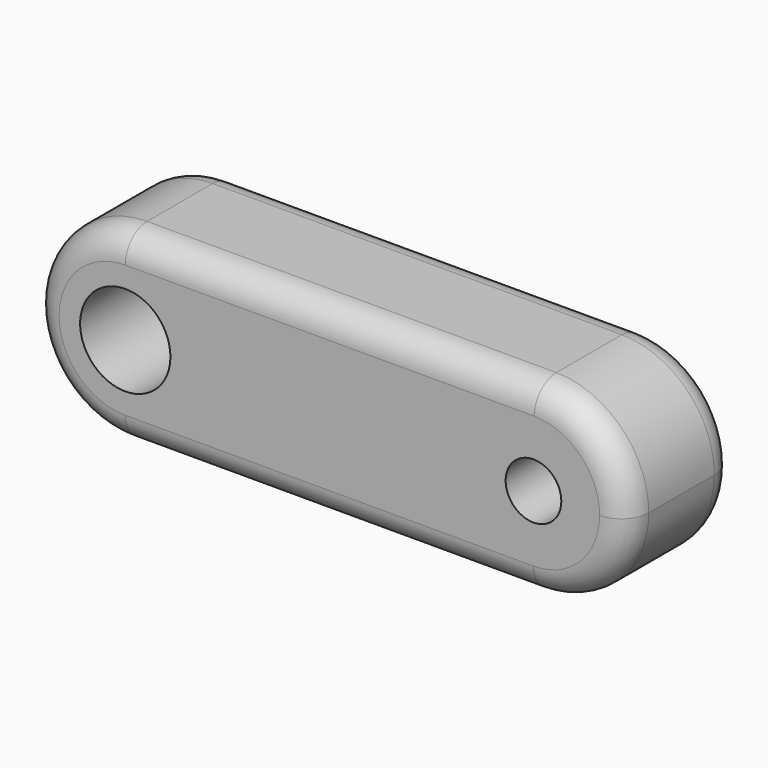
from build123d import *

# Parameters (mm, degrees)
F0_R     = 8.3978836091
F0_R_2   = 5.1785228726
F1_DEPTH = 25.4
F2_R     = 5.08
F3_R     = 5.08


with BuildPart() as f1:
    # F0 (on Front) → F1 (new body)
    with BuildSketch(Plane.XZ):
        with BuildLine():
            ThreePointArc((0, -17.3770133917), (12.2874040061, -12.2874040061), (17.3770133917, 0))
            ThreePointArc((17.3770133917, 0), (12.2874040061, 12.2874040061), (0, 17.3770133917))
            ThreePointArc((0, 17.3770133917), (-17.3770133917, 0), (0, -17.3770133917))
        make_face()
        Circle(F0_R, mode=Mode.SUBTRACT)
        with BuildLine():
            ThreePointArc((0, 17.3770133917), (12.2874040061, 12.2874040061), (17.3770133917, 0))
            ThreePointArc((17.3770133917, 0), (12.2874040061, -12.2874040061), (0, -17.3770133917))
            Line((0, -17.3770133917), (75.9285844538, -17.3780516278))
            ThreePointArc((75.9285844538, -17.3780516278), (58.5510294425, -0.0948615367), (75.7388642212, 17.3770133917))
            Line((75.7388642212, 17.3770133917), (0, 17.3770133917))
        make_face()
        with BuildLine():
            Line((76.1187800984, 17.3770133917), (75.7388642212, 17.3770133917))
            ThreePointArc((75.7388642212, 17.3770133917), (58.5510294425, -0.0948615367), (75.9285844538, -17.3780516278))
            ThreePointArc((75.9285844538, -17.3780516278), (88.2168762687, -12.2882221924), (93.3068737892, 0))
            ThreePointArc((93.3068737892, 0), (88.2839380495, 12.220793337), (76.1187800984, 17.3770133917))
        make_face()
        with Locations((75.9288221598, 0)):
            Circle(F0_R_2, mode=Mode.SUBTRACT)
    extrude(amount=F1_DEPTH)

    # F2
    f2_edges = [f1.edges().sort_by_distance(p)[0] for p in [
        (-17.377013, -25.4, 0),
        (38.05939, -25.4, 17.377013),
        (93.306614, -25.4, -0.095099),
        (37.964292, -25.4, -17.377533),
    ]]
    fillet(f2_edges, radius=F2_R)

    # F3
    f3_edges = [f1.edges().sort_by_distance(p)[0] for p in [
        (-17.377013, 0, 0),
        (37.964292, 0, -17.377533),
        (93.306614, 0, -0.095099),
        (38.05939, 0, 17.377013),
    ]]
    fillet(f3_edges, radius=F3_R)


solid = f1.part
